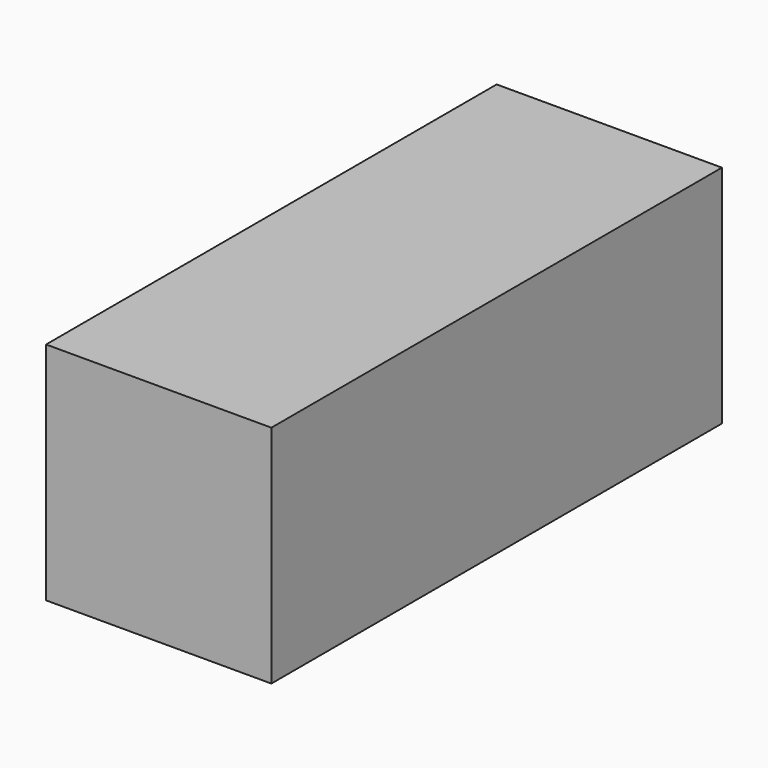
from build123d import *

# Parameters (mm, degrees)
F5_W          = 200
F5_H          = 500
F6_DEPTH      = 100
F6_DEPTH_BACK = 100


# Not quite as in the source:
# - a feature of the source that left no trace in its solid (it failed there, or was rolled back) is left out
# - the program builds the solid bodies; features that only make, move or delete a surface that nothing else refers to are left out


with BuildPart() as f6:
    # F5 (on Top) → F6 (new body, two sides)
    with BuildSketch(Plane.XY) as f6_sk:
        Rectangle(F5_W, F5_H)
    extrude(amount=F6_DEPTH)
    extrude(f6_sk.sketch, amount=-F6_DEPTH_BACK)


solid = f6.part
